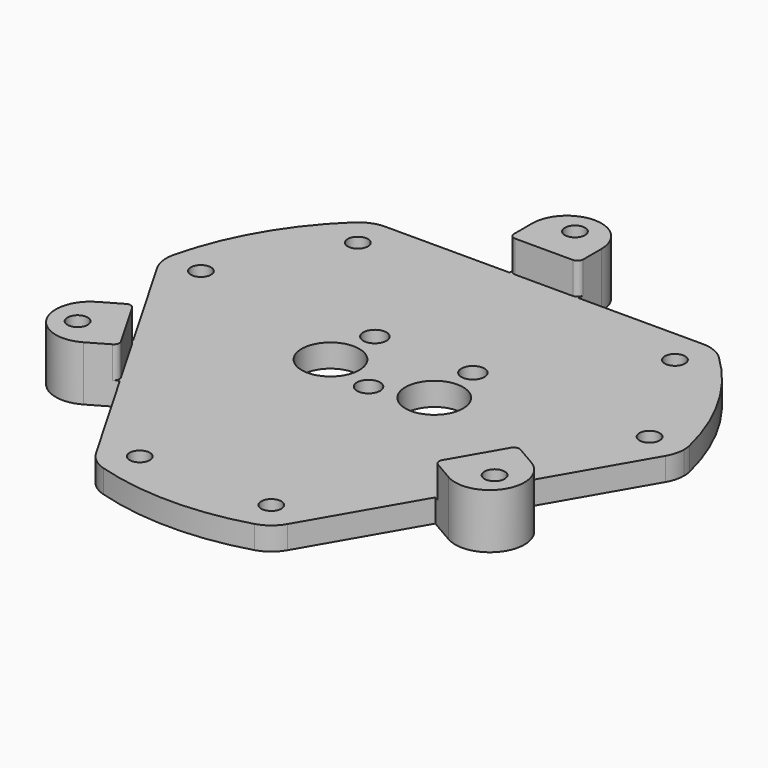
from build123d import *

# Parameters (mm, degrees)
F0_W     = 30
F0_H     = 18
F0_R     = 2
F0_R_2   = 5
F0_R_3   = 1.75
F1_DEPTH = 4
F2_DEPTH = 5.5
F3_R     = 1


# Not quite as in the source:
# - a feature names something its author has since deleted; it is built from what else it names


with BuildPart() as f1:
    # F0 (on Top) → F1 (new body)
    with BuildSketch(Plane.XY):
        with BuildLine():
            ThreePointArc((-32.905765, 9.292011), (-37.35285, 3.496456), (-44.101917, 6.292011))
            Line((-44.101917, 6.292011), (-33.351917, -12.327535))
            Line((-33.351917, -12.327535), (-27.351917, -22.71984))
            Line((-27.351917, -22.71984), (-16.601917, -41.339386))
            ThreePointArc((-16.601917, -41.339386), (-12.958679, -32.543831), (-5.405765, -38.339386))
            ThreePointArc((-5.405765, -38.339386), (-7.818648, -43.149022), (-13.11663, -44.090294))
            ThreePointArc((-13.11663, -44.090294), (0, -46), (13.116629, -44.090294))
            ThreePointArc((13.116629, -44.090294), (6.596129, -34.752269), (17.405765, -38.339386))
            ThreePointArc((17.405765, -38.339386), (17.20132, -39.8923), (16.601917, -41.339386))
            Line((16.601917, -41.339386), (27.351917, -22.71984))
            Line((27.351917, -22.71984), (33.351917, -12.327535))
            Line((33.351917, -12.327535), (44.101917, 6.292011))
            ThreePointArc((44.101917, 6.292011), (32.968364, 10.156462), (44.741629, 10.685813))
            ThreePointArc((44.741629, 10.685813), (39.837169, 23), (31.625, 33.404481))
            ThreePointArc((31.625, 33.404481), (33.011352, 31.419083), (33.5, 29.047375))
            ThreePointArc((33.5, 29.047375), (23.257359, 24.804734), (27.5, 35.047375))
            Line((27.5, 35.047375), (6, 35.047375))
            Line((6, 35.047375), (-6, 35.047375))
            Line((-6, 35.047375), (-27.5, 35.047375))
            ThreePointArc((-27.5, 35.047375), (-23.257359, 33.290016), (-21.5, 29.047375))
            ThreePointArc((-21.5, 29.047375), (-29.871708, 23.536023), (-31.625, 33.404481))
            ThreePointArc((-31.625, 33.404481), (-39.837169, 23), (-44.741629, 10.685813))
            ThreePointArc((-44.741629, 10.685813), (-38.204048, 15.250836), (-32.905765, 9.292011))
        make_face()
        with Locations((0, 3)):
            Rectangle(F0_W, F0_H, mode=Mode.SUBTRACT)
        with Locations((0, 3)):
            Rectangle(F0_W, F0_H)
        with Locations((0, -3)):
            Circle(F0_R, mode=Mode.SUBTRACT)
        with Locations((-9, 0)):
            Circle(F0_R_2, mode=Mode.SUBTRACT)
        with Locations((-8.5, 9)):
            Circle(F0_R, mode=Mode.SUBTRACT)
        with Locations((9, 0)):
            Circle(F0_R_2, mode=Mode.SUBTRACT)
        with Locations((8.5, 9)):
            Circle(F0_R, mode=Mode.SUBTRACT)
        with BuildLine():
            ThreePointArc((6, 40), (4.242641, 44.242641), (0, 46))
            ThreePointArc((0, 46), (-4.242641, 44.242641), (-6, 40))
            Line((-6, 40), (-6, 35.047375))
            Line((-6, 35.047375), (6, 35.047375))
            Line((6, 35.047375), (6, 40))
        make_face()
        with Locations((0, 41.75)):
            Circle(F0_R_3, mode=Mode.SUBTRACT)
        with BuildLine():
            Line((-27.351917, -22.71984), (-33.351917, -12.327535))
            Line((-33.351917, -12.327535), (-37.641016, -14.803848))
            ThreePointArc((-37.641016, -14.803848), (-40.436571, -18.447086), (-39.837169, -23))
            ThreePointArc((-39.837169, -23), (-36.19393, -25.795555), (-31.641016, -25.196152))
            Line((-31.641016, -25.196152), (-27.351917, -22.71984))
        make_face()
        with Locations((-36.156561, -20.875)):
            Circle(F0_R_3, mode=Mode.SUBTRACT)
        with BuildLine():
            ThreePointArc((31.641016, -25.196152), (36.19393, -25.795555), (39.837168, -23.000001))
            ThreePointArc((39.837168, -23.000001), (40.436571, -18.447086), (37.641016, -14.803848))
            Line((37.641016, -14.803848), (33.351917, -12.327535))
            Line((33.351917, -12.327535), (27.351917, -22.71984))
            Line((27.351917, -22.71984), (31.641016, -25.196152))
        make_face()
        with Locations((36.156561, -20.875)):
            Circle(F0_R_3, mode=Mode.SUBTRACT)
        with BuildLine():
            ThreePointArc((-44.741629, 10.685813), (-44.843165, 8.42756), (-44.101917, 6.292011))
            ThreePointArc((-44.101917, 6.292011), (-37.35285, 3.496456), (-32.905765, 9.292011))
            ThreePointArc((-32.905765, 9.292011), (-38.204048, 15.250836), (-44.741629, 10.685813))
        make_face()
        with Locations((-38.905765, 9.292011)):
            Circle(F0_R_3, mode=Mode.SUBTRACT)
        with BuildLine():
            ThreePointArc((-27.5, 35.047375), (-29.720063, 34.62154), (-31.625, 33.404481))
            ThreePointArc((-31.625, 33.404481), (-29.871708, 23.536023), (-21.5, 29.047375))
            ThreePointArc((-21.5, 29.047375), (-23.257359, 33.290016), (-27.5, 35.047375))
        make_face()
        with Locations((-27.5, 29.047375)):
            Circle(F0_R_3, mode=Mode.SUBTRACT)
        with BuildLine():
            ThreePointArc((33.5, 29.047375), (33.011352, 31.419083), (31.625, 33.404481))
            ThreePointArc((31.625, 33.404481), (29.720063, 34.62154), (27.5, 35.047375))
            ThreePointArc((27.5, 35.047375), (23.257359, 24.804734), (33.5, 29.047375))
        make_face()
        with Locations((27.5, 29.047375)):
            Circle(F0_R_3, mode=Mode.SUBTRACT)
        with BuildLine():
            ThreePointArc((44.905765, 9.292011), (44.86459, 9.993728), (44.741629, 10.685813))
            ThreePointArc((44.741629, 10.685813), (32.968364, 10.156462), (44.101917, 6.292011))
            ThreePointArc((44.101917, 6.292011), (44.70132, 7.739097), (44.905765, 9.292011))
        make_face()
        with Locations((38.905765, 9.292011)):
            Circle(F0_R_3, mode=Mode.SUBTRACT)
        with BuildLine():
            ThreePointArc((17.405765, -38.339386), (6.596129, -34.752269), (13.116629, -44.090294))
            ThreePointArc((13.116629, -44.090294), (15.123102, -43.0491), (16.601917, -41.339386))
            ThreePointArc((16.601917, -41.339386), (17.20132, -39.8923), (17.405765, -38.339386))
        make_face()
        with Locations((11.405765, -38.339386)):
            Circle(F0_R_3, mode=Mode.SUBTRACT)
        with BuildLine():
            ThreePointArc((-16.601917, -41.339386), (-15.123102, -43.0491), (-13.11663, -44.090294))
            ThreePointArc((-13.11663, -44.090294), (-7.818648, -43.149022), (-5.405765, -38.339386))
            ThreePointArc((-5.405765, -38.339386), (-12.958679, -32.543831), (-16.601917, -41.339386))
        make_face()
        with Locations((-11.405765, -38.339386)):
            Circle(F0_R_3, mode=Mode.SUBTRACT)
    extrude(amount=-F1_DEPTH)

    # F0 (on Top) → F2 (join)
    with BuildSketch(Plane.XY):
        with BuildLine():
            Line((-27.351917, -22.71984), (-33.351917, -12.327535))
            Line((-33.351917, -12.327535), (-37.641016, -14.803848))
            ThreePointArc((-37.641016, -14.803848), (-40.436571, -18.447086), (-39.837169, -23))
            ThreePointArc((-39.837169, -23), (-36.19393, -25.795555), (-31.641016, -25.196152))
            Line((-31.641016, -25.196152), (-27.351917, -22.71984))
        make_face()
        with Locations((-36.156561, -20.875)):
            Circle(F0_R_3, mode=Mode.SUBTRACT)
        with BuildLine():
            ThreePointArc((6, 40), (4.242641, 44.242641), (0, 46))
            ThreePointArc((0, 46), (-4.242641, 44.242641), (-6, 40))
            Line((-6, 40), (-6, 35.047375))
            Line((-6, 35.047375), (6, 35.047375))
            Line((6, 35.047375), (6, 40))
        make_face()
        with Locations((0, 41.75)):
            Circle(F0_R_3, mode=Mode.SUBTRACT)
        with BuildLine():
            ThreePointArc((31.641016, -25.196152), (36.19393, -25.795555), (39.837168, -23.000001))
            ThreePointArc((39.837168, -23.000001), (40.436571, -18.447086), (37.641016, -14.803848))
            Line((37.641016, -14.803848), (33.351917, -12.327535))
            Line((33.351917, -12.327535), (27.351917, -22.71984))
            Line((27.351917, -22.71984), (31.641016, -25.196152))
        make_face()
        with Locations((36.156561, -20.875)):
            Circle(F0_R_3, mode=Mode.SUBTRACT)
    extrude(amount=F2_DEPTH)

    # F3
    f3_edges = [f1.edges().sort_by_distance(p)[0] for p in [
        (6, 35.047375, 2.75),
        (-6, 35.047375, 2.75),
        (33.351917, -12.327535, 2.75),
        (27.351917, -22.71984, 2.75),
        (-33.351917, -12.327535, 2.75),
        (-27.351917, -22.71984, 2.75),
    ]]
    fillet(f3_edges, radius=F3_R)


solid = f1.part
